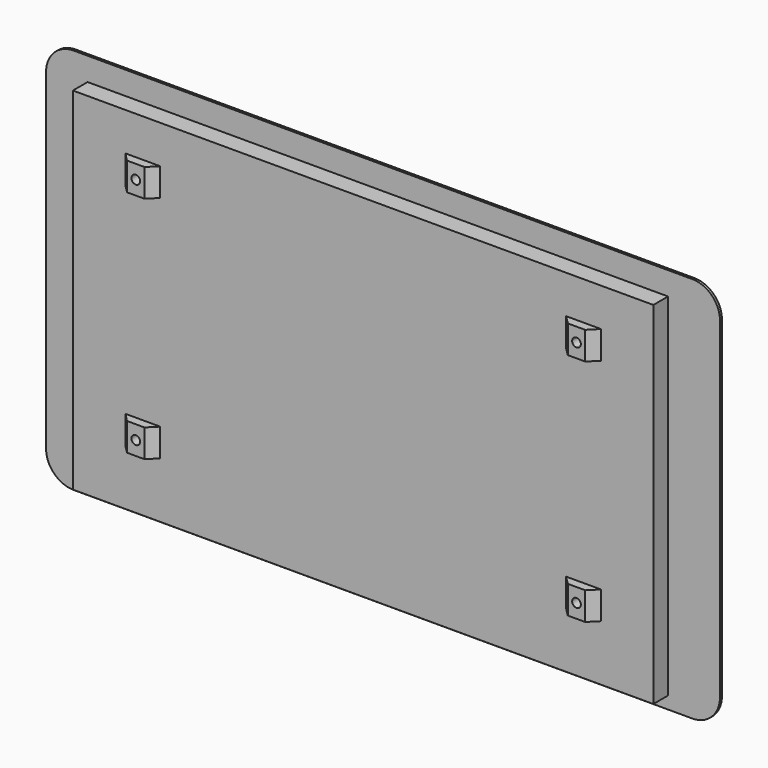
from build123d import *

# Parameters (mm, degrees)
F0_W         = 166.2
F0_H         = 100.6
F1_DEPTH     = 5.96
F2_DEPTH     = 0.7
F3_W         = 15
F3_H         = 8
F4_DEPTH     = 2.5
F5_T4_DEPTH  = 33.7168298797
F5_T9_DEPTH  = 33.7168298797
F5_T14_DEPTH = 33.7168298797
F5_T19_DEPTH = 33.7168298797
F5_T24_DEPTH = 33.7168298797
F5_T29_DEPTH = 33.7168298797
F5_T34_DEPTH = 33.7168298797
F5_T39_DEPTH = 33.7168298797
F6_D         = 2.5
F6_DEPTH     = 2.501


# Not quite as in the source:
# - a fillet or chamfer that OpenCascade refuses, or shapes differently, is made with other operations: its cross-section is extruded or revolved along the edge and cut away or added


with BuildPart() as f1:
    # F0 (on Front) → F1 (new body)
    with BuildSketch(Plane.XZ):
        with Locations((-1.49, -1.55)):
            Rectangle(F0_W, F0_H)
    extrude(amount=F1_DEPTH)

    # F0 (on Front) → F2 (join)
    with BuildSketch(Plane.XZ):
        with BuildLine():
            ThreePointArc((-96.48, -47.5), (-94.1720014358, -53.0720014358), (-88.6, -55.38))
            Line((-88.6, -55.38), (88.6, -55.38))
            ThreePointArc((88.6, -55.38), (94.1720014357, -53.0720014357), (96.48, -47.5))
            Line((96.48, -47.5), (96.48, 47.5))
            ThreePointArc((96.48, 47.5), (94.1720014358, 53.0720014358), (88.6, 55.38))
            Line((88.6, 55.38), (-88.6, 55.38))
            ThreePointArc((-88.6, 55.38), (-94.1720014357, 53.0720014357), (-96.48, 47.5))
            Line((-96.48, 47.5), (-96.48, -47.5))
        make_face()
        with Locations((-1.49, -1.55)):
            Rectangle(F0_W, F0_H, mode=Mode.SUBTRACT)
    extrude(amount=F2_DEPTH)

    # F3 (on face) → F4 (join)
    with BuildSketch(Plane.XZ.offset(5.96)):
        with Locations((-64.59, 33.8)):
            Rectangle(F3_W, F3_H)
        with Locations((-64.59, -31.85)):
            Rectangle(F3_W, F3_H)
        with Locations((61.61, -31.85)):
            Rectangle(F3_W, F3_H)
        with Locations((61.61, 33.8)):
            Rectangle(F3_W, F3_H)
    extrude(amount=F4_DEPTH)

    # F5: chamfer of 5 on 8 edges, made by hand


with BuildPart() as f5_tool2:
    # F5_s3 → F5_t4 (new body)
    with BuildSketch(Plane.XY.offset(50.6584149398)):
        Polygon((-72.09, -3.46), (-67.09, -8.46), (-72.09, -8.46), align=None)
    extrude(amount=-F5_T4_DEPTH)

    split(bisect_by=Plane.XZ.offset(5.96), keep=Keep.TOP)


with BuildPart() as f1_1:
    add(f1.part)

    # F5_t1: cut F5_tool2
    add(f5_tool2.part, mode=Mode.SUBTRACT)


with BuildPart() as f5_tool7:
    # F5_s8 → F5_t9 (new body)
    with BuildSketch(Plane.XY.offset(16.9415850602)):
        Polygon((-57.09, -3.46), (-62.09, -8.46), (-57.09, -8.46), align=None)
    extrude(amount=F5_T9_DEPTH)

    split(bisect_by=Plane.XZ.offset(5.96), keep=Keep.TOP)


with BuildPart() as f1_2:
    add(f1_1.part)

    # F5_t6: cut F5_tool7
    add(f5_tool7.part, mode=Mode.SUBTRACT)


with BuildPart() as f5_tool12:
    # F5_s13 → F5_t14 (new body)
    with BuildSketch(Plane.XY.offset(-14.9915850602)):
        Polygon((-72.09, -3.46), (-67.09, -8.46), (-72.09, -8.46), align=None)
    extrude(amount=-F5_T14_DEPTH)

    split(bisect_by=Plane.XZ.offset(5.96), keep=Keep.TOP)


with BuildPart() as f1_3:
    add(f1_2.part)

    # F5_t11: cut F5_tool12
    add(f5_tool12.part, mode=Mode.SUBTRACT)


with BuildPart() as f5_tool17:
    # F5_s18 → F5_t19 (new body)
    with BuildSketch(Plane.XY.offset(-48.7084149398)):
        Polygon((-57.09, -3.46), (-62.09, -8.46), (-57.09, -8.46), align=None)
    extrude(amount=F5_T19_DEPTH)

    split(bisect_by=Plane.XZ.offset(5.96), keep=Keep.TOP)


with BuildPart() as f1_4:
    add(f1_3.part)

    # F5_t16: cut F5_tool17
    add(f5_tool17.part, mode=Mode.SUBTRACT)


with BuildPart() as f5_tool22:
    # F5_s23 → F5_t24 (new body)
    with BuildSketch(Plane.XY.offset(50.6584149398)):
        Polygon((54.11, -3.46), (59.11, -8.46), (54.11, -8.46), align=None)
    extrude(amount=-F5_T24_DEPTH)

    split(bisect_by=Plane.XZ.offset(5.96), keep=Keep.TOP)


with BuildPart() as f1_5:
    add(f1_4.part)

    # F5_t21: cut F5_tool22
    add(f5_tool22.part, mode=Mode.SUBTRACT)


with BuildPart() as f5_tool27:
    # F5_s28 → F5_t29 (new body)
    with BuildSketch(Plane.XY.offset(16.9415850602)):
        Polygon((69.11, -3.46), (64.11, -8.46), (69.11, -8.46), align=None)
    extrude(amount=F5_T29_DEPTH)

    split(bisect_by=Plane.XZ.offset(5.96), keep=Keep.TOP)


with BuildPart() as f1_6:
    add(f1_5.part)

    # F5_t26: cut F5_tool27
    add(f5_tool27.part, mode=Mode.SUBTRACT)


with BuildPart() as f5_tool32:
    # F5_s33 → F5_t34 (new body)
    with BuildSketch(Plane.XY.offset(-14.9915850602)):
        Polygon((54.11, -3.46), (59.11, -8.46), (54.11, -8.46), align=None)
    extrude(amount=-F5_T34_DEPTH)

    split(bisect_by=Plane.XZ.offset(5.96), keep=Keep.TOP)


with BuildPart() as f1_7:
    add(f1_6.part)

    # F5_t31: cut F5_tool32
    add(f5_tool32.part, mode=Mode.SUBTRACT)


with BuildPart() as f5_tool37:
    # F5_s38 → F5_t39 (new body)
    with BuildSketch(Plane.XY.offset(-48.7084149398)):
        Polygon((69.11, -3.46), (64.11, -8.46), (69.11, -8.46), align=None)
    extrude(amount=F5_T39_DEPTH)

    split(bisect_by=Plane.XZ.offset(5.96), keep=Keep.TOP)


with BuildPart() as f1_8:
    add(f1_7.part)

    # F5_t36: cut F5_tool37
    add(f5_tool37.part, mode=Mode.SUBTRACT)

    # F6 (through all, one way)
    with BuildSketch(Plane(origin=(0, -5.96, 0), x_dir=(1, 0, 0), z_dir=(0, 1, 0))):
        with Locations((-64.59, -33.8), (-64.59, 31.85), (61.61, 31.85), (61.61, -33.8)):
            Circle(F6_D / 2)
    extrude(amount=-F6_DEPTH, mode=Mode.SUBTRACT)


solid = f1_8.part
